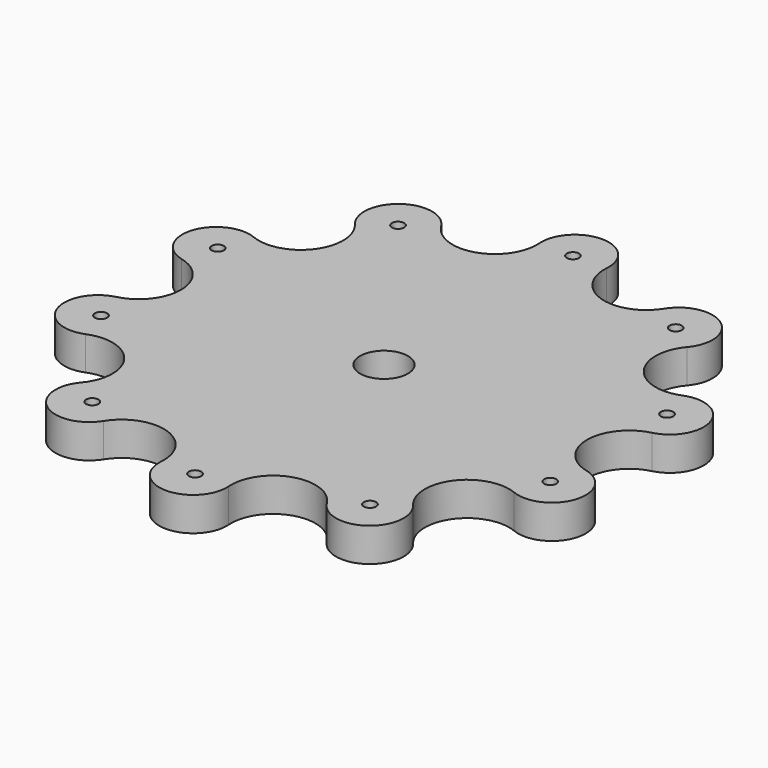
from build123d import *

# Parameters (mm, degrees)
F0_R            = 19.416407865
F1_DEPTH        = 2.75
F3_DEPTH        = 2.75
F3_COPIES_COUNT = 10
F5_DEPTH        = 25
F5_COPIES_COUNT = 10
F6_R            = 1.9472144129
F7_DEPTH        = 25
F8_R            = 0.5
F9_DEPTH        = 25
F9_COPIES_COUNT = 10


# Not quite as in the source:
# - a pattern or mirror of a feature is missing from the dataset's text; its kind, count and spacing are read off the source's solid


with BuildPart() as f1:
    # F0 (on Top) → F1 (new body)
    with BuildSketch(Plane.XY):
        Circle(F0_R)
    extrude(amount=-F1_DEPTH)

    # F2 (on face) → F3 (join)
    with BuildSketch(Plane.XY):
        with BuildLine():
            ThreePointArc((-2.7430957606, 19.22166278), (0, 19.416407865), (2.7430957606, 19.22166278))
            ThreePointArc((2.7430957606, 19.22166278), (0, 22.166407865), (-2.7430957606, 19.22166278))
        make_face()
    f3 = extrude(amount=-F3_DEPTH)

    # F3_copies: F3 ×10 about axis
    f3_copies_axis = Axis((0, 0, 0), (0, 0, 1))
    for i in range(1, F3_COPIES_COUNT):
        add(f3.rotate(f3_copies_axis, i * 360 / F3_COPIES_COUNT))

    # F4 (on face) → F5 (cut)
    with BuildSketch(Plane.XY):
        with BuildLine():
            Line((-6.2381998898, 19.1992051025), (-9.0789988191, 17.1630030829))
            ThreePointArc((-9.0789988191, 17.1630030829), (-5.1059656467, 15.7145464123), (-2.7430957606, 19.22166278))
            Line((-2.7430957606, 19.22166278), (-6.2381998898, 19.1992051025))
        make_face()
    f5 = extrude(amount=-F5_DEPTH, mode=Mode.SUBTRACT)

    # F5_copies: F5 ×10 about axis
    f5_copies_axis = Axis((0, 0, 0), (0, 0, 1))
    for i in range(1, F5_COPIES_COUNT):
        add(f5.rotate(f5_copies_axis, i * 360 / F5_COPIES_COUNT), mode=Mode.SUBTRACT)

    # F6 (on face) → F7 (cut)
    with BuildSketch(Plane.XY):
        Circle(F6_R)
    extrude(amount=-F7_DEPTH, mode=Mode.SUBTRACT)

    # F8 (on face) → F9 (cut)
    with BuildSketch(Plane.XY):
        with Locations((0, 19.2206762207)):
            Circle(F8_R)
    f9 = extrude(amount=-F9_DEPTH, mode=Mode.SUBTRACT)

    # F9_copies: F9 ×10 about axis
    f9_copies_axis = Axis((0, 0, 0), (0, 0, 1))
    for i in range(1, F9_COPIES_COUNT):
        add(f9.rotate(f9_copies_axis, i * 360 / F9_COPIES_COUNT), mode=Mode.SUBTRACT)


solid = f1.part
